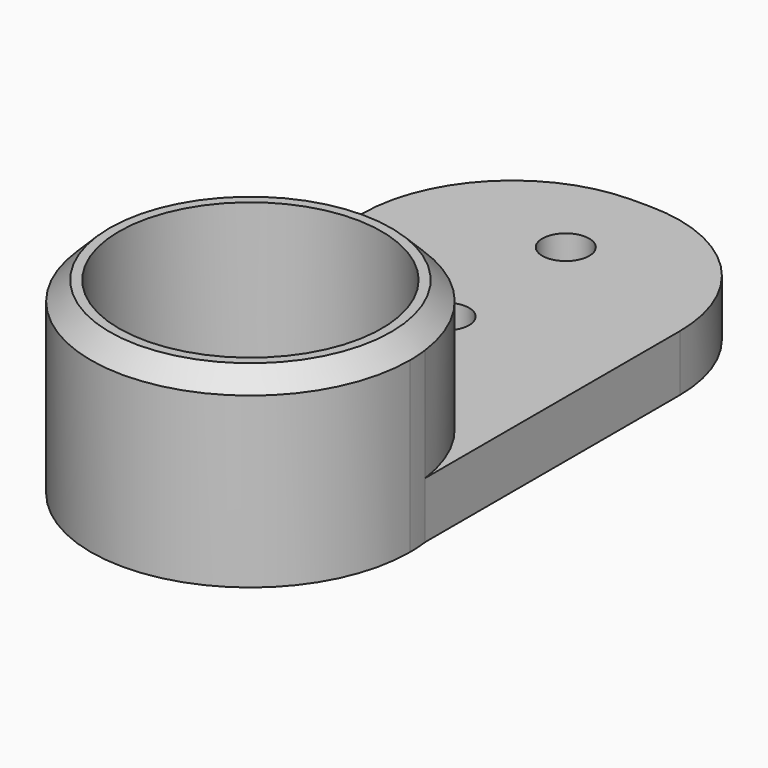
from build123d import *

# Parameters (mm, degrees)
F1_DEPTH = 10
F2_DEPTH = 3
F3_R     = 8
F4_D     = 14
F6_D     = 2.5


# Not quite as in the source:
# - a fillet or chamfer that OpenCascade refuses, or shapes differently, is made with other operations: its cross-section is extruded or revolved along the edge and cut away or added


with BuildPart() as f1:
    # F0 (on Top) → F1 (new body)
    with BuildSketch(Plane.XY):
        with BuildLine():
            ThreePointArc((8.4283100441, 1.101630519), (-0.5519803552, 8.482058576), (-8.5, 0))
            Line((-8.5, 0), (8.4283100441, 0))
            Line((8.4283100441, 0), (8.4283100441, 1.101630519))
        make_face()
        with BuildLine():
            Line((8.4283100441, 0), (-8.5, 0))
            ThreePointArc((-8.5, 0), (0, -8.5), (8.5, 0))
            ThreePointArc((8.5, 0), (8.482058576, 0.5519803552), (8.4283100441, 1.101630519))
            Line((8.4283100441, 1.101630519), (8.4283100441, 0))
        make_face()
    extrude(amount=F1_DEPTH)

    # F0 (on Top) → F2 (join)
    with BuildSketch(Plane.XY):
        with BuildLine():
            Line((-8.5, 26.0569844395), (-8.5, 0))
            ThreePointArc((-8.5, 0), (-0.5519803552, 8.482058576), (8.4283100441, 1.101630519))
            Line((8.4283100441, 1.101630519), (8.4283100441, 26.0569844395))
            Line((8.4283100441, 26.0569844395), (-8.5, 26.0569844395))
        make_face()
    extrude(amount=F2_DEPTH)

    # F3
    f3_edges = [f1.edges().sort_by_distance(p)[0] for p in [
        (-8.5, 26.056984, 1.5),
        (8.42831, 26.056984, 1.5),
    ]]
    fillet(f3_edges, radius=F3_R)

    # F4 (through all)
    with Locations(Plane(origin=(0, 0, 0), x_dir=(1, 0, 0), z_dir=(0, 0, -1))):
        with Locations((0, 0)):
            Hole(F4_D / 2)

    # F5: chamfer of 1 on 1 edges, made by hand

    # F5_s1 → F5_t2 (revolve, cut)
    with BuildSketch(Plane.XZ):
        Polygon((-8.5, 9), (-7.5, 10), (-8.5, 10), align=None)
    revolve(axis=Axis((0, 0, 10), (0, 0, 1)), mode=Mode.SUBTRACT)

    # F6 (through all)
    with Locations(Plane(origin=(0, 0, 0), x_dir=(1, 0, 0), z_dir=(0, 0, -1))):
        with Locations((0, -21), (0, -13)):
            Hole(F6_D / 2)


solid = f1.part
